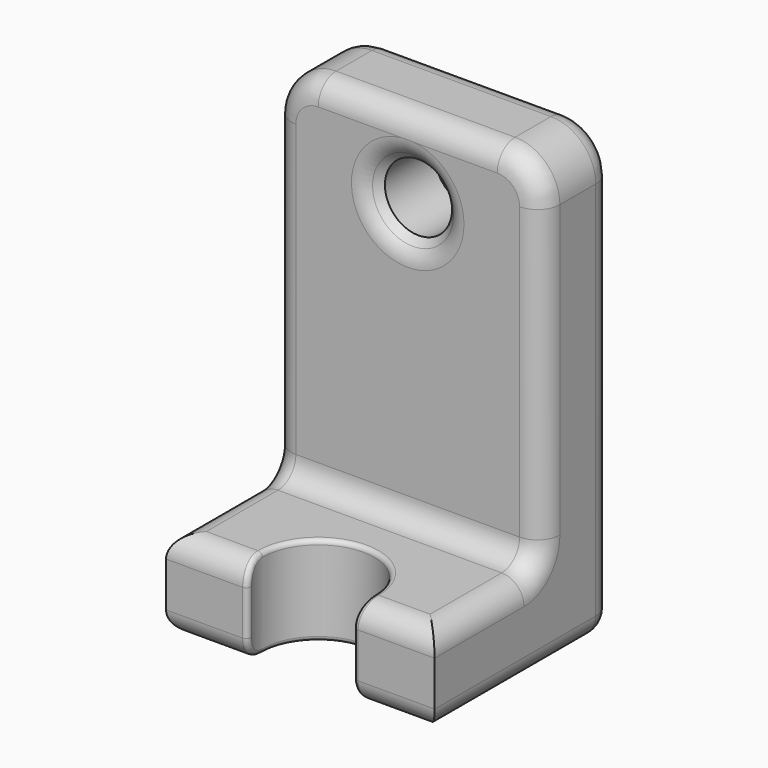
from build123d import *

# Parameters (mm, degrees)
F0_R         = 7.5
F1_DEPTH     = 20
F2_SIZE      = 3
F3_W         = 60
F3_H         = 20
F4_DEPTH     = 30
F5_T1_DEPTH  = 60
F5_T3_DEPTH  = 65
F5_T5_DEPTH  = 40
F5_T7_DEPTH  = 37.5
F5_T9_DEPTH  = 85
F5_T12_ANGLE = 90
F5_T14_ANGLE = 90
F5_T18_ANGLE = 90
F5_T20_ANGLE = 90
F6_T1_DEPTH  = 40
F6_T3_DEPTH  = 85
F6_T5_DEPTH  = 50
F6_T7_DEPTH  = 57.5
F6_T9_DEPTH  = 85
F6_S13_W     = 5
F6_S13_H     = 5
F6_T14_DEPTH = 5
F6_S19_W     = 5
F6_S19_H     = 5
F6_T20_DEPTH = 5
F6_T26_ANGLE = 90
F6_T28_ANGLE = 90
F8_DEPTH     = 20.001
F9_R         = 1


# Not quite as in the source:
# - a fillet or chamfer that OpenCascade refuses, or shapes differently, is made with other operations: its cross-section is extruded or revolved along the edge and cut away or added


with BuildPart() as f1:
    # F0 (on Front) → F1 (new body)
    with BuildSketch(Plane.XZ):
        with BuildLine():
            Line((20, 50), (-20, 50))
            ThreePointArc((-20, 50), (-27.0710678119, 47.0710678119), (-30, 40))
            Line((-30, 40), (-30, -50))
            Line((-30, -50), (30, -50))
            Line((30, -50), (30, 40))
            ThreePointArc((30, 40), (27.0710678119, 47.0710678119), (20, 50))
        make_face()
        with Locations((0, 32.5)):
            Circle(F0_R, mode=Mode.SUBTRACT)
    extrude(amount=F1_DEPTH)

    # F2
    f2_edges = [f1.edges().sort_by_distance(p)[0] for p in [
        (7.5, -10, 32.5),
        (-7.5, 0, 32.5),
        (-7.5, -20, 32.5),
    ]]
    chamfer(f2_edges, length=F2_SIZE)

    # F3 (on face) → F4 (join)
    with BuildSketch(Plane.XZ.offset(20)):
        with Locations((0, -40)):
            Rectangle(F3_W, F3_H)
    extrude(amount=F4_DEPTH)

    # F5: fillet of radius 5 on 10 edges, made by hand

    # F5_s2 → F5_t1 (join)
    with BuildSketch(Plane.YZ.offset(-30)):
        with BuildLine():
            ThreePointArc((-20, -25), (-21.4644660941, -28.5355339059), (-25, -30))
            Line((-25, -30), (-20, -30))
            Line((-20, -30), (-20, -25))
        make_face()
    extrude(amount=F5_T1_DEPTH)

    # F5_s4 → F5_t3 (cut)
    with BuildSketch(Plane.XY.offset(-25)):
        with BuildLine():
            ThreePointArc((25, -20), (28.5355339059, -18.5355339059), (30, -15))
            Line((30, -15), (30, -20))
            Line((30, -20), (25, -20))
        make_face()
        with BuildLine():
            ThreePointArc((-25, -20), (-28.5355339059, -18.5355339059), (-30, -15))
            Line((-30, -15), (-30, -20))
            Line((-30, -20), (-25, -20))
        make_face()
    extrude(amount=F5_T3_DEPTH, mode=Mode.SUBTRACT)

    # F5_s6 → F5_t5 (cut)
    with BuildSketch(Plane.YZ.offset(-20)):
        with BuildLine():
            ThreePointArc((-20, 45), (-18.5355339059, 48.5355339059), (-15, 50))
            Line((-15, 50), (-20, 50))
            Line((-20, 50), (-20, 45))
        make_face()
    extrude(amount=F5_T5_DEPTH, mode=Mode.SUBTRACT)

    # F5_s8 → F5_t7 (cut)
    with BuildSketch(Plane.XZ.offset(25)):
        with BuildLine():
            ThreePointArc((30, -35), (28.5355339059, -31.4644660941), (25, -30))
            Line((25, -30), (30, -30))
            Line((30, -30), (30, -35))
        make_face()
        with BuildLine():
            ThreePointArc((-30, -35), (-28.5355339059, -31.4644660941), (-25, -30))
            Line((-25, -30), (-30, -30))
            Line((-30, -30), (-30, -35))
        make_face()
    extrude(amount=F5_T7_DEPTH, mode=Mode.SUBTRACT)

    # F5_s10 → F5_t9 (cut)
    with BuildSketch(Plane.YZ.offset(-42.5)):
        with BuildLine():
            ThreePointArc((-45, -30), (-48.5355339059, -31.4644660941), (-50, -35))
            Line((-50, -35), (-50, -30))
            Line((-50, -30), (-45, -30))
        make_face()
    extrude(amount=F5_T9_DEPTH, mode=Mode.SUBTRACT)

    # F5_s11 → F5_t12 (revolve, cut)
    with BuildSketch(Plane.XY.offset(40)):
        with BuildLine():
            ThreePointArc((25, -20), (28.5355339059, -18.5355339059), (30, -15))
            Line((30, -15), (30, -20))
            Line((30, -20), (25, -20))
        make_face()
    revolve(axis=Axis((20, -20, 40), (0, -1, 0)), revolution_arc=F5_T12_ANGLE, mode=Mode.SUBTRACT)

    # F5_s13 → F5_t14 (revolve, cut)
    with BuildSketch(Plane.YZ.offset(-20)):
        with BuildLine():
            ThreePointArc((-20, 45), (-18.5355339059, 48.5355339059), (-15, 50))
            Line((-15, 50), (-20, 50))
            Line((-20, 50), (-20, 45))
        make_face()
    revolve(axis=Axis((-20, -20, 40), (0, -1, 0)), revolution_arc=F5_T14_ANGLE, mode=Mode.SUBTRACT)

    # F5_s15 → F5_t16 (revolve, cut)
    with BuildSketch(Plane.XY.offset(32.5)):
        with BuildLine():
            ThreePointArc((9.0355339059, -18.5355339059), (10.65765065, -19.6193976626), (12.5710678119, -20))
            Line((12.5710678119, -20), (10.5, -20))
            Line((10.5, -20), (9.0355339059, -18.5355339059))
        make_face()
    revolve(axis=Axis((0, -20, 32.5), (0, -1, 0)), mode=Mode.SUBTRACT)

    # F5_s17 → F5_t18 (revolve, cut)
    with BuildSketch(Plane.XY.offset(-25)):
        with BuildLine():
            ThreePointArc((-30, -15), (-28.5355339059, -18.5355339059), (-25, -20))
            Line((-25, -20), (-30, -20))
            Line((-30, -20), (-30, -15))
        make_face()
    revolve(axis=Axis((-30, -25, -25), (-1, 0, 0)), revolution_arc=F5_T18_ANGLE, mode=Mode.SUBTRACT)

    # F5_s19 → F5_t20 (revolve, cut)
    with BuildSketch(Plane.XY.offset(-25)):
        with BuildLine():
            ThreePointArc((30, -15), (28.5355339059, -18.5355339059), (25, -20))
            Line((25, -20), (30, -20))
            Line((30, -20), (30, -15))
        make_face()
    revolve(axis=Axis((30, -25, -25), (-1, 0, 0)), revolution_arc=F5_T20_ANGLE, mode=Mode.SUBTRACT)

    # F6: fillet of radius 5 on 10 edges, made by hand

    # F6_s2 → F6_t1 (cut)
    with BuildSketch(Plane.YZ.offset(-20)):
        with BuildLine():
            ThreePointArc((0, 45), (-1.4644660941, 48.5355339059), (-5, 50))
            Line((-5, 50), (0, 50))
            Line((0, 50), (0, 45))
        make_face()
    extrude(amount=F6_T1_DEPTH, mode=Mode.SUBTRACT)

    # F6_s4 → F6_t3 (cut)
    with BuildSketch(Plane.XY.offset(-45)):
        with BuildLine():
            ThreePointArc((-25, 0), (-28.5355339059, -1.4644660941), (-30, -5))
            Line((-30, -5), (-30, 0))
            Line((-30, 0), (-25, 0))
        make_face()
        with BuildLine():
            ThreePointArc((25, 0), (28.5355339059, -1.4644660941), (30, -5))
            Line((30, -5), (30, 0))
            Line((30, 0), (25, 0))
        make_face()
    extrude(amount=F6_T3_DEPTH, mode=Mode.SUBTRACT)

    # F6_s6 → F6_t5 (cut)
    with BuildSketch(Plane.YZ.offset(-25)):
        with BuildLine():
            ThreePointArc((0, -45), (-1.4644660941, -48.5355339059), (-5, -50))
            Line((-5, -50), (0, -50))
            Line((0, -50), (0, -45))
        make_face()
    extrude(amount=F6_T5_DEPTH, mode=Mode.SUBTRACT)

    # F6_s8 → F6_t7 (cut)
    with BuildSketch(Plane.XZ.offset(5)):
        with BuildLine():
            ThreePointArc((-30, -45), (-28.5355339059, -48.5355339059), (-25, -50))
            Line((-25, -50), (-30, -50))
            Line((-30, -50), (-30, -45))
        make_face()
        with BuildLine():
            ThreePointArc((25, -50), (28.5355339059, -48.5355339059), (30, -45))
            Line((30, -45), (30, -50))
            Line((30, -50), (25, -50))
        make_face()
    extrude(amount=F6_T7_DEPTH, mode=Mode.SUBTRACT)

    # F6_s10 → F6_t9 (cut)
    with BuildSketch(Plane.YZ.offset(-42.5)):
        with BuildLine():
            ThreePointArc((-45, -50), (-48.5355339059, -48.5355339059), (-50, -45))
            Line((-50, -45), (-50, -50))
            Line((-50, -50), (-45, -50))
        make_face()
    extrude(amount=F6_T9_DEPTH, mode=Mode.SUBTRACT)


with BuildPart() as f6_tool12:
    # F6_s13 → F6_t14 (new body)
    with BuildSketch(Plane.XY.offset(-45)):
        with Locations((-27.5, -2.5)):
            Rectangle(F6_S13_W, F6_S13_H)
    extrude(amount=-F6_T14_DEPTH)

    # F6_s15 → F6_t16 (revolve, cut)
    with BuildSketch(Plane(origin=(-25, -5, -45), x_dir=(0.7071067812, -0.7071067812, 0), z_dir=(0.7071067812, 0.7071067812, 0))):
        with BuildLine():
            ThreePointArc((0, -5), (5, 0), (0, 5))
            Line((0, 5), (0, -5))
        make_face()
    revolve(axis=Axis((-25, -5, -45), (0, 0, -1)), mode=Mode.SUBTRACT)


with BuildPart() as f1_1:
    add(f1.part)

    # F6_t11: cut F6_tool12
    add(f6_tool12.part, mode=Mode.SUBTRACT)


with BuildPart() as f6_tool18:
    # F6_s19 → F6_t20 (new body)
    with BuildSketch(Plane.XY.offset(-45)):
        with Locations((27.5, -2.5)):
            Rectangle(F6_S19_W, F6_S19_H)
    extrude(amount=-F6_T20_DEPTH)

    # F6_s21 → F6_t22 (revolve, cut)
    with BuildSketch(Plane(origin=(25, -5, -45), x_dir=(-0.7071067812, -0.7071067812, 0), z_dir=(0.7071067812, -0.7071067812, 0))):
        with BuildLine():
            ThreePointArc((0, -5), (5, 0), (0, 5))
            Line((0, 5), (0, -5))
        make_face()
    revolve(axis=Axis((25, -5, -45), (0, 0, -1)), mode=Mode.SUBTRACT)


with BuildPart() as f1_2:
    add(f1_1.part)

    # F6_t17: cut F6_tool18
    add(f6_tool18.part, mode=Mode.SUBTRACT)

    # F6_s23 → F6_t24 (revolve, cut)
    with BuildSketch(Plane.XY.offset(32.5)):
        with BuildLine():
            ThreePointArc((9.0355339059, -1.4644660941), (10.65765065, -0.3806023374), (12.5710678119, 0))
            Line((12.5710678119, 0), (10.5, 0))
            Line((10.5, 0), (9.0355339059, -1.4644660941))
        make_face()
    revolve(axis=Axis((0, 0, 32.5), (0, -1, 0)), mode=Mode.SUBTRACT)

    # F6_s25 → F6_t26 (revolve, cut)
    with BuildSketch(Plane.YZ.offset(-20)):
        with BuildLine():
            ThreePointArc((0, 45), (-1.4644660941, 48.5355339059), (-5, 50))
            Line((-5, 50), (0, 50))
            Line((0, 50), (0, 45))
        make_face()
    revolve(axis=Axis((-20, 0, 40), (0, -1, 0)), revolution_arc=F6_T26_ANGLE, mode=Mode.SUBTRACT)

    # F6_s27 → F6_t28 (revolve, cut)
    with BuildSketch(Plane.XY.offset(40)):
        with BuildLine():
            ThreePointArc((25, 0), (28.5355339059, -1.4644660941), (30, -5))
            Line((30, -5), (30, 0))
            Line((30, 0), (25, 0))
        make_face()
    revolve(axis=Axis((20, 0, 40), (0, -1, 0)), revolution_arc=F6_T28_ANGLE, mode=Mode.SUBTRACT)

    # F7 (on face) → F8 (cut, through all)
    with BuildSketch(Plane.XY.offset(-30)):
        with BuildLine():
            Line((-12.5, -45), (12.5, -45))
            ThreePointArc((12.5, -45), (0, -32.5), (-12.5, -45))
        make_face()
        with BuildLine():
            ThreePointArc((-12.5, -45), (0, -57.5), (12.5, -45))
            Line((12.5, -45), (-12.5, -45))
        make_face()
    extrude(amount=-F8_DEPTH, mode=Mode.SUBTRACT)

    # F9
    f9_edges = [f1_2.edges().sort_by_distance(p)[0] for p in [
        (0, -32.5, -50),
        (-11.98926, -48.536614, -48.534454),
        (-11.456439, -50, -40),
        (-11.98926, -48.536614, -31.465546),
        (0, -32.5, -30),
        (11.98926, -48.536614, -31.465546),
        (11.456439, -50, -40),
        (11.98926, -48.536614, -48.534454),
    ]]
    fillet(f9_edges, radius=F9_R)


solid = f1_2.part
